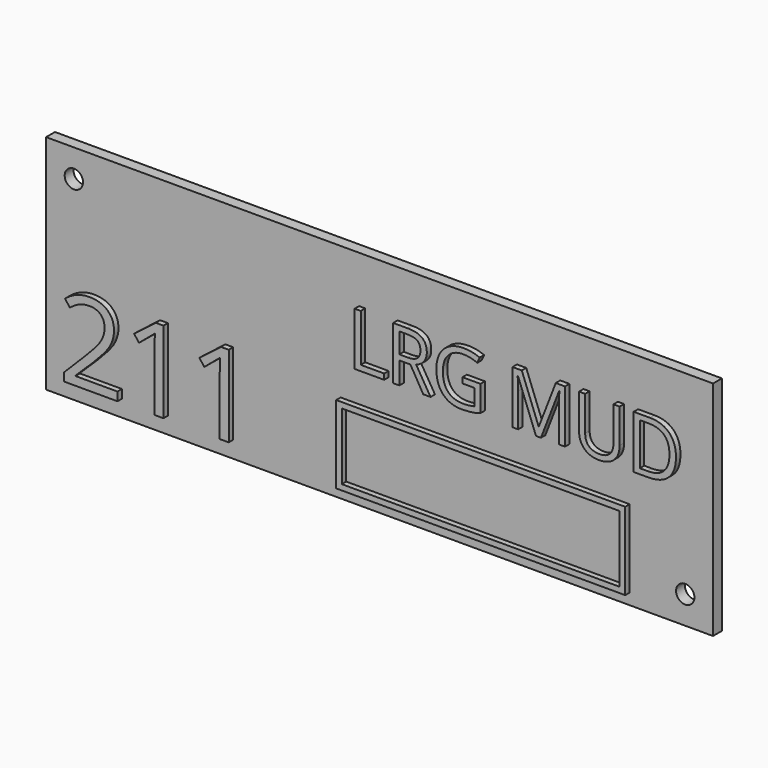
from build123d import *

# Parameters (mm, degrees)
F0_W         = 120
F0_H         = 40
F1_DEPTH     = 2
F3_D         = 3.3
F4_TEXT_SIZE = 13.3672155115
F5_DEPTH     = 1
F6_TEXT_SIZE = 20.5478077656
F7_DEPTH     = 1
F8_W         = 52
F8_H         = 14
F8_W_2       = 49.99999962
F8_H_2       = 11.99999962
F9_DEPTH     = 1


# Not quite as in the source:
# - Text() gives the source's letters only with a copy of the font that has no kerning and outlines rounded to 1/6400 em; it was checked with that copy


with BuildPart() as f1:
    # F0 (on Front) → F1 (new body)
    with BuildSketch(Plane.XZ):
        Rectangle(F0_W, F0_H)
    extrude(amount=F1_DEPTH)

    # F3 (through all)
    with Locations(Plane.XZ.offset(2)):
        with Locations((-55, 15), (55, -15)):
            Hole(F3_D / 2)

    # F4 (on face) → F5 (join)
    with BuildSketch(Plane.XZ.offset(2)):
        with Locations((-5, 2)):
            Text('LRG MUD', F4_TEXT_SIZE, font='Open Sans', text_align=(TextAlign.LEFT, TextAlign.BOTTOM))
    extrude(amount=F5_DEPTH)

    # F6 (on face) → F7 (join)
    with BuildSketch(Plane.XZ.offset(2)):
        with Locations((-57, -17)):
            Text('211', F6_TEXT_SIZE, font='Open Sans', text_align=(TextAlign.LEFT, TextAlign.BOTTOM))
    extrude(amount=F7_DEPTH)

    # F8 (on face) → F9 (join)
    with BuildSketch(Plane.XZ.offset(2)):
        with Locations((19, -11)):
            Rectangle(F8_W, F8_H)
        with Locations((19, -11)):
            Rectangle(F8_W_2, F8_H_2, mode=Mode.SUBTRACT)
    extrude(amount=F9_DEPTH)


solid = f1.part
